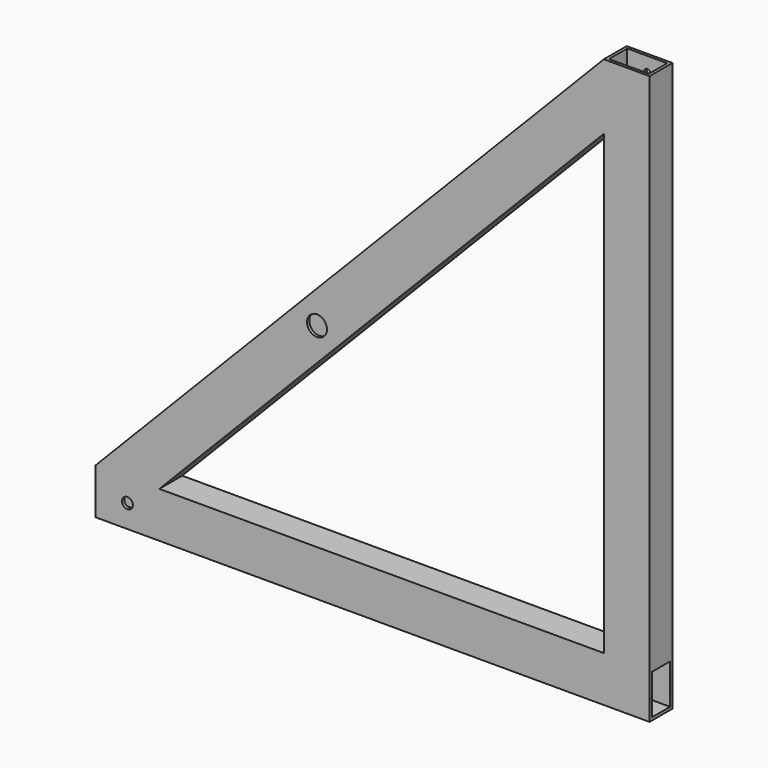
from build123d import *

# Parameters (mm, degrees)
F0_W         = 50
F0_H         = 80
F0_W_2       = 40
F0_H_2       = 70
F1_DEPTH     = 969
F2_W         = 80
F2_H         = 50
F2_W_2       = 70
F2_H_2       = 40
F3_DEPTH     = 914.4
F5_DEPTH     = 50
F6_R         = 17.5
F6_R_2       = 9.5
F7_DEPTH     = 50.001
F8_T         = 5
F8_T3_DEPTH  = 60
F8_T5_DEPTH  = 979
F8_T7_DEPTH  = 924.4
F8_T9_DEPTH  = 80
F8_T11_DEPTH = 50
F9_START     = -25.4
F6_R_3       = 5
F9_DEPTH     = 27.432


# Not quite as in the source:
# - a shell that OpenCascade refuses in one call is made with other operations: the cavity is built on its own and cut out


with BuildPart() as f1:
    # F0 (on Right) → F1 (new body)
    with BuildSketch(Plane.YZ):
        with Locations((-25, 40)):
            Rectangle(F0_W, F0_H)
        with Locations((-25, 40)):
            Rectangle(F0_W_2, F0_H_2, mode=Mode.SUBTRACT)
    extrude(amount=-F1_DEPTH)

    # F2 (on face) → F3 (join)
    with BuildSketch(Plane.XY.offset(80)):
        with Locations((-40, -25)):
            Rectangle(F2_W, F2_H)
        with Locations((-40, -25)):
            Rectangle(F2_W_2, F2_H_2, mode=Mode.SUBTRACT)
    extrude(amount=F3_DEPTH)

    # F4 (on face) → F5 (join)
    with BuildSketch(Plane.XZ.offset(50)):
        Polygon((-80, 994.4), (-969, 80), (-857.4231981277, 80), (-80, 879.6352895028), align=None)
    extrude(amount=-F5_DEPTH)

    # F6 (on face) → F7 (cut, through all)
    with BuildSketch(Plane.XZ.offset(50)):
        with Locations((-581.6838212861, 421)):
            Circle(F6_R)
        with Locations((-913.2115990639, 40)):
            Circle(F6_R_2)
    extrude(amount=-F7_DEPTH, mode=Mode.SUBTRACT)

    # F8: shell of thickness 5, made by hand


with BuildPart() as f8_core1:
    # F8_t2: copy of F1
    add(f1.part)

    # the walls: a layer under each face that stays
    f8_faces = [f8_core1.faces().sort_by_distance(p)[0] for p in [
        (-484.5, -25, 0),
        (-484.5, -50, 497.2),
        (-484.5, 0, 497.2),
        (0, -25, 497.2),
        (-969, -46.4285714286, 5.7142857143),
        (-524.5, -25, 537.2),
        (-74.2857142857, -46.4285714286, 994.4),
        (-922.7115990639, -47.5, 40),
        (-468.7115990639, -25, 80),
        (-80, -25, 479.8176447514),
        (-468.7115990639, -25, 479.8176447514),
        (-922.7115990639, -2.5, 40),
        (-484.5, -25, 75),
        (-484.5, -5, 40),
        (-484.5, -25, 5),
        (-484.5, -45, 40),
        (-40, -5, 537.2),
        (-5, -25, 537.2),
        (-40, -45, 537.2),
        (-75, -25, 537.2),
        (-40, -25, 80),
    ]]
    thicken(f8_faces, amount=-F8_T, mode=Mode.SUBTRACT)

    # F8_s4 → F8_t3 (cut)
    with BuildSketch(Plane.XZ.offset(-5)):
        Polygon((-80.05, 80.05), (-80, 75), (-75, 75), (-75, 80), align=None)
        Polygon((-857.3873483818, 80.0151460803), (-857.4231981277, 75), (-869.2578593558, 75), (-861.0081727218, 83.4853919665), align=None)
        Polygon((-80.0141502541, 879.6004355831), (-75, 879.6352895028), (-75, 891.9509410517), (-83.5849745941, 883.1206814692), align=None)
    extrude(amount=F8_T3_DEPTH, mode=Mode.SUBTRACT)

    # F8_s6 → F8_t5 (cut)
    with BuildSketch(Plane.YZ.offset(-974)):
        Polygon((-44.95, 74.95), (-45, 80), (-50, 80), (-50, 75), align=None)
        Polygon((-5.05, 74.95), (-5, 80), (0, 80), (0, 75), align=None)
        Polygon((-5.05, 5.05), (0, 5), (0, 0), (-5, 0), align=None)
        Polygon((-44.95, 5.05), (-45, 0), (-50, 0), (-50, 5), align=None)
    extrude(amount=F8_T5_DEPTH, mode=Mode.SUBTRACT)

    # F8_s8 → F8_t7 (cut)
    with BuildSketch(Plane.XY.offset(75)):
        Polygon((-74.95, -5.05), (-75, 0), (-80, 0), (-80, -5), align=None)
        Polygon((-5.05, -5.05), (-5, 0), (0, 0), (0, -5), align=None)
        Polygon((-5.05, -44.95), (0, -45), (0, -50), (-5, -50), align=None)
        Polygon((-74.95, -44.95), (-75, -50), (-80, -50), (-80, -45), align=None)
    extrude(amount=F8_T7_DEPTH, mode=Mode.SUBTRACT)

    # F8_s10 → F8_t9 (cut)
    with BuildSketch(Plane.YZ.offset(-80)):
        Polygon((-5.05, 80.05), (0, 80), (0, 75), (-5, 75), align=None)
        Polygon((-44.95, 80.05), (-50, 80), (-50, 75), (-45, 75), align=None)
    extrude(amount=F8_T9_DEPTH, mode=Mode.SUBTRACT)

    # F8_s12 → F8_t11 (cut)
    with BuildSketch(Plane.XZ):
        Polygon((-5.05, 80.05), (0, 80), (0, 75), (-5, 75), align=None)
        Polygon((-74.95, 80.05), (-80, 80), (-80, 75), (-75, 75), align=None)
    extrude(amount=F8_T11_DEPTH, mode=Mode.SUBTRACT)


with BuildPart() as f1_1:
    add(f1.part)

    # what is left inside the walls is the cavity
    f8_cavity = [f8_core1.part.solids().sort_by_distance(p)[0] for p in [
        (-635.349987, -5.05, 363.508502),
    ]]
    add(f8_cavity, mode=Mode.SUBTRACT)

    # F6 (on face) → F9 (cut)
    with BuildSketch(Plane.XZ.offset(50).offset(F9_START)):
        with Locations((-40, 969.4)):
            Circle(F6_R_3)
        with Locations((-40, 944.4)):
            Circle(F6_R_3)
    extrude(amount=-F9_DEPTH, mode=Mode.SUBTRACT)


solid = f1_1.part
